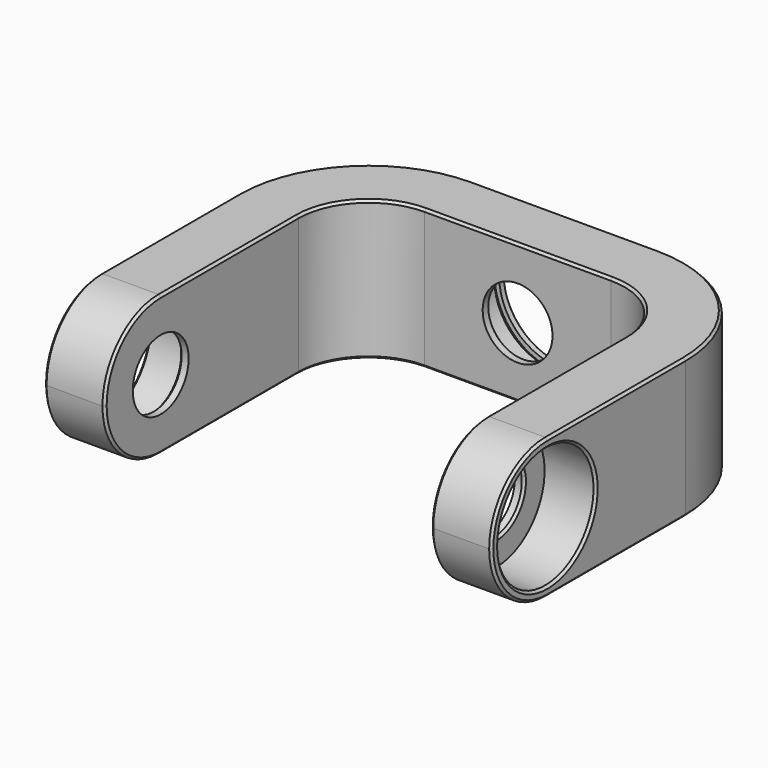
from build123d import *

# Parameters (mm, degrees)
F0_W          = 30
F0_H          = 13
F0_W_2        = 13
F0_H_2        = 30
F1_DEPTH      = 15
F1_DEPTH_BACK = 15
F2_R          = 14.99999
F3_R          = 28
F4_R          = 12.995
F4_R_2        = 7.5
F5_DEPTH      = 11
F6_DEPTH      = 13
F7_R          = 12.995
F7_R_2        = 7.5
F8_DEPTH      = 11
F9_DEPTH      = 13
F10_START     = -1.7
F7_R_3        = 14
F10_DEPTH     = 1.3
F12_SIZE      = 0.5


# Not quite as in the source:
# - a fillet or chamfer is up to 0.001 mm smaller than in the source, because OpenCascade refuses the exact size


with BuildPart() as f1:
    # F0 (on Top) → F1 (new body, two sides)
    with BuildSketch(Plane.XY) as f1_sk:
        with Locations((0, 58.5)):
            Rectangle(F0_W, F0_H)
        Polygon((-48, 15), (-35, 15), (-35, 52), (-15, 52), (-15, 65), (-48, 65), align=None)
        with Locations((-41.5, 0)):
            Rectangle(F0_W_2, F0_H_2)
        Polygon((35, 52), (35, 15), (48, 15), (48, 65), (15, 65), (15, 52), align=None)
        with Locations((41.5, 0)):
            Rectangle(F0_W_2, F0_H_2)
    extrude(amount=F1_DEPTH)
    extrude(f1_sk.sketch, amount=-F1_DEPTH_BACK)

    # F2 (radius 15 in the source; OpenCascade refuses exactly that, so slightly less here)
    f2_edges = [f1.edges().sort_by_distance(p)[0] for p in [
        (-41.5, -15, 15),
        (-41.5, -15, -15),
        (41.5, -15, 15),
        (41.5, -15, -15),
        (-35, 52, 0),
        (35, 52, 0),
    ]]
    fillet(f2_edges, radius=F2_R)

    # F3
    f3_edges = [f1.edges().sort_by_distance(p)[0] for p in [
        (48, 65, 0),
        (-48, 65, 0),
    ]]
    fillet(f3_edges, radius=F3_R)

    # F4 (on face) → F5 (cut)
    with BuildSketch(Plane(origin=(-48, 0, 0), x_dir=(0, -1, 0), z_dir=(-1, 0, 0))):
        Circle(F4_R)
        Circle(F4_R_2, mode=Mode.SUBTRACT)
        Circle(F4_R_2)
    extrude(amount=-F5_DEPTH, mode=Mode.SUBTRACT)

    # F4 (on face) → F6 (cut)
    with BuildSketch(Plane(origin=(-48, 0, 0), x_dir=(0, -1, 0), z_dir=(-1, 0, 0))):
        Circle(F4_R_2)
    extrude(amount=-F6_DEPTH, mode=Mode.SUBTRACT)

    # F7 (on face) → F8 (cut)
    with BuildSketch(Plane(origin=(0, 65, 0), x_dir=(-1, 0, 0), z_dir=(0, 1, 0))):
        Circle(F7_R)
        Circle(F7_R_2, mode=Mode.SUBTRACT)
        Circle(F7_R_2)
    extrude(amount=-F8_DEPTH, mode=Mode.SUBTRACT)

    # F7 (on face) → F9 (cut)
    with BuildSketch(Plane(origin=(0, 65, 0), x_dir=(-1, 0, 0), z_dir=(0, 1, 0))):
        Circle(F7_R_2)
    extrude(amount=-F9_DEPTH, mode=Mode.SUBTRACT)

    # F7 (on face) → F10 (cut)
    with BuildSketch(Plane(origin=(0, 65, 0), x_dir=(-1, 0, 0), z_dir=(0, 1, 0)).offset(F10_START)):
        Circle(F7_R_3)
        Circle(F7_R, mode=Mode.SUBTRACT)
    extrude(amount=-F10_DEPTH, mode=Mode.SUBTRACT)

    # F11: F1 across plane


with BuildPart() as f1_1:
    add(f1.part)
    add(f1.part.mirror(Plane.YZ), mode=Mode.INTERSECT)

    # F12
    f12_edges = [f1_1.edges().sort_by_distance(p)[0] for p in [
        (-30.606605, 47.606605, 15),
        (0, 65, -15),
        (-48, 12.995, 0),
        (-37, 7.5, 0),
        (48, 12.995, 0),
        (37, 7.5, 0),
        (12.995, 65, 0),
        (7.5, 54, 0),
        (-48, 18.499995, 15),
        (-48, -10.606605, 10.606605),
        (-48, 18.499995, -15),
        (-48, -15, 0),
        (-48, -10.606605, -10.606605),
        (-35, 18.5, 15),
        (-35, -10.606605, 10.606605),
        (-35, -15, 0),
        (-35, 18.5, -15),
        (-35, -10.606605, -10.606605),
        (-30.606605, 47.606605, -15),
        (0, 52, 15),
        (0, 52, -15),
        (0, 65, 15),
        (39.79899, 56.79899, 15),
        (39.79899, 56.79899, -15),
        (48, 18.499995, 15),
        (48, -10.606605, 10.606605),
        (48, -15, 0),
        (48, 18.499995, -15),
        (48, -10.606605, -10.606605),
        (35, 18.5, 15),
        (35, -10.606605, 10.606605),
        (35, 18.5, -15),
        (35, -15, 0),
        (35, -10.606605, -10.606605),
        (30.606605, 47.606605, -15),
        (30.606605, 47.606605, 15),
        (-39.79899, 56.79899, -15),
        (-39.79899, 56.79899, 15),
    ]]
    chamfer(f12_edges, length=F12_SIZE)


solid = f1_1.part
